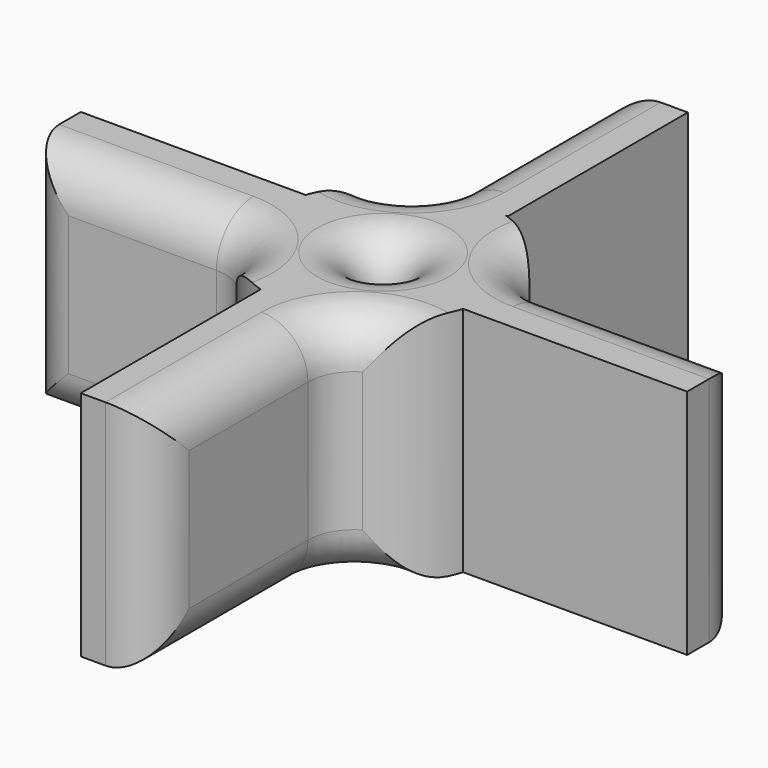
from build123d import *

# Parameters (mm, degrees)
F0_R         = 4.211
F0_W         = 0.5461883944
F0_H         = 48.4801451702
F1_DEPTH     = 25
F2_T1_DEPTH  = 50
F2_T3_DEPTH  = 100
F2_T5_DEPTH  = 67.0975783302
F2_T7_DEPTH  = 67.2386600166
F2_T9_DEPTH  = 67.0975783302
F2_T11_DEPTH = 66.9249549756
F2_T18_ANGLE = 202.5983722588
F2_T20_ANGLE = 202.5983722588
F2_T22_ANGLE = 202.6248548609
F2_T24_ANGLE = 202.6248548609
F2_T26_ANGLE = 201.5951809175
F2_T28_ANGLE = 201.5951809175
F2_T30_ANGLE = 202.6248548609
F2_T32_ANGLE = 202.6248548609


# Not quite as in the source:
# - a fillet or chamfer that OpenCascade refuses, or shapes differently, is made with other operations: its cross-section is extruded or revolved along the edge and cut away or added


with BuildPart() as f1:
    # F0 (on Top) → F1 (new body, symmetric)
    with BuildSketch(Plane.XY):
        with BuildLine():
            Line((7.6582201656, -71.9089287116), (7.6582201656, -23.4287835415))
            ThreePointArc((7.6582201656, -23.4287835415), (17.4241101733, -17.4343516945), (23.4242794808, -7.6719857367))
            Line((23.4242794808, -7.6719857367), (71.7281472729, -7.6719857367))
            Line((71.7281472729, -7.6719857367), (71.7281472729, 8.1906429889))
            Line((71.7281472729, 8.1906429889), (23.2480021027, 8.1906429889))
            ThreePointArc((23.2480021027, 8.1906429889), (17.2293028181, 17.6268930541), (7.6582201656, 23.4287835415))
            Line((7.6582201656, 23.4287835415), (7.6582201656, 71.9089287116))
            Line((7.6582201656, 71.9089287116), (-7.6582201656, 71.9089287116))
            Line((-7.6582201656, 71.9089287116), (-7.6582201656, 23.4287835415))
            ThreePointArc((-7.6582201656, 23.4287835415), (-17.2293028181, 17.6268930541), (-23.2480021027, 8.1906429889))
            Line((-23.2480021027, 8.1906429889), (-71.7281472729, 8.1906429889))
            Line((-71.7281472729, 8.1906429889), (-71.7281472729, -7.6719857367))
            Line((-71.7281472729, -7.6719857367), (-23.4242794808, -7.6719857367))
            ThreePointArc((-23.4242794808, -7.6719857367), (-17.4241101733, -17.4343516945), (-7.6582201656, -23.4287835415))
            Line((-7.6582201656, -23.4287835415), (-7.6582201656, -71.9089287116))
            Line((-7.6582201656, -71.9089287116), (7.6582201656, -71.9089287116))
        make_face()
        Circle(F0_R, mode=Mode.SUBTRACT)
        with Locations((7.9313143628, 47.6688561266)):
            Rectangle(F0_W, F0_H)
    extrude(amount=F1_DEPTH, both=True)

    # F2: fillet of radius 10 on 18 edges, made by hand

    # F2_s2 → F2_t1 (join)
    with BuildSketch(Plane.XY.offset(-25)):
        with BuildLine():
            ThreePointArc((-12.5618550278, 21.2074522892), (-8.9701924441, 24.8597673709), (-7.6582201656, 29.8113503815))
            Line((-7.6582201656, 29.8113503815), (-7.6582201656, 23.4287835415))
            ThreePointArc((-7.6582201656, 23.4287835415), (-10.170862222, 22.4523895387), (-12.5618550278, 21.2074522892))
        make_face()
        with BuildLine():
            ThreePointArc((20.9784825584, 12.9406145096), (24.6161046934, 9.458510237), (29.4894872562, 8.1906429889))
            Line((29.4894872562, 8.1906429889), (23.2480021027, 8.1906429889))
            ThreePointArc((23.2480021027, 8.1906429889), (22.2404146484, 10.6263912316), (20.9784825584, 12.9406145096))
        make_face()
        with BuildLine():
            ThreePointArc((12.5618550278, -21.2074522892), (8.9701924441, -24.8597673709), (7.6582201656, -29.8113503815))
            Line((7.6582201656, -29.8113503815), (7.6582201656, -23.4287835415))
            ThreePointArc((7.6582201656, -23.4287835415), (10.170862222, -22.4523895387), (12.5618550278, -21.2074522892))
        make_face()
        with BuildLine():
            ThreePointArc((-21.2016487218, -12.5716476969), (-24.8536155677, -8.9828148787), (-29.8031922973, -7.6719857367))
            Line((-29.8031922973, -7.6719857367), (-23.4242794808, -7.6719857367))
            ThreePointArc((-23.4242794808, -7.6719857367), (-22.4470496684, -10.1826418734), (-21.2016487218, -12.5716476969))
        make_face()
    extrude(amount=F2_T1_DEPTH)

    # F2_s4 → F2_t3 (cut)
    with BuildSketch(Plane.XY.offset(-50)):
        with BuildLine():
            ThreePointArc((2.3417798344, 71.9089287116), (-4.7292879775, 68.9799965235), (-7.6582201656, 61.9089287116))
            Line((-7.6582201656, 61.9089287116), (-7.6582201656, 71.9089287116))
            Line((-7.6582201656, 71.9089287116), (2.3417798344, 71.9089287116))
        make_face()
        with BuildLine():
            ThreePointArc((71.7281472729, -1.8093570111), (68.7992150847, 5.2617108008), (61.7281472729, 8.1906429889))
            Line((61.7281472729, 8.1906429889), (71.7281472729, 8.1906429889))
            Line((71.7281472729, 8.1906429889), (71.7281472729, -1.8093570111))
        make_face()
        with BuildLine():
            ThreePointArc((-2.3417798344, -71.9089287116), (4.7292879775, -68.9799965235), (7.6582201656, -61.9089287116))
            Line((7.6582201656, -61.9089287116), (7.6582201656, -71.9089287116))
            Line((7.6582201656, -71.9089287116), (-2.3417798344, -71.9089287116))
        make_face()
        with BuildLine():
            ThreePointArc((-71.7281472729, 2.3280142633), (-68.7992150847, -4.7430535485), (-61.7281472729, -7.6719857367))
            Line((-61.7281472729, -7.6719857367), (-71.7281472729, -7.6719857367))
            Line((-71.7281472729, -7.6719857367), (-71.7281472729, 2.3280142633))
        make_face()
    extrude(amount=F2_T3_DEPTH, mode=Mode.SUBTRACT)

    # F2_s6 → F2_t5 (cut)
    with BuildSketch(Plane.XZ.offset(-96.9089287116)):
        with BuildLine():
            ThreePointArc((2.3417798344, -25), (-4.7292879775, -22.0710678119), (-7.6582201656, -15))
            Line((-7.6582201656, -15), (-7.6582201656, -25))
            Line((-7.6582201656, -25), (2.3417798344, -25))
        make_face()
        with BuildLine():
            ThreePointArc((2.3417798344, 25), (-4.7292879775, 22.0710678119), (-7.6582201656, 15))
            Line((-7.6582201656, 15), (-7.6582201656, 25))
            Line((-7.6582201656, 25), (2.3417798344, 25))
        make_face()
    extrude(amount=F2_T5_DEPTH, mode=Mode.SUBTRACT)

    # F2_s8 → F2_t7 (cut)
    with BuildSketch(Plane.YZ.offset(29.4894872562)):
        with BuildLine():
            ThreePointArc((-1.8093570111, -25), (5.2617108008, -22.0710678119), (8.1906429889, -15))
            Line((8.1906429889, -15), (8.1906429889, -25))
            Line((8.1906429889, -25), (-1.8093570111, -25))
        make_face()
        with BuildLine():
            ThreePointArc((-1.8093570111, 25), (5.2617108008, 22.0710678119), (8.1906429889, 15))
            Line((8.1906429889, 15), (8.1906429889, 25))
            Line((8.1906429889, 25), (-1.8093570111, 25))
        make_face()
    extrude(amount=F2_T7_DEPTH, mode=Mode.SUBTRACT)

    # F2_s10 → F2_t9 (cut)
    with BuildSketch(Plane.XZ.offset(29.8113503815)):
        with BuildLine():
            ThreePointArc((-2.3417798344, -25), (4.7292879775, -22.0710678119), (7.6582201656, -15))
            Line((7.6582201656, -15), (7.6582201656, -25))
            Line((7.6582201656, -25), (-2.3417798344, -25))
        make_face()
        with BuildLine():
            ThreePointArc((-2.3417798344, 25), (4.7292879775, 22.0710678119), (7.6582201656, 15))
            Line((7.6582201656, 15), (7.6582201656, 25))
            Line((7.6582201656, 25), (-2.3417798344, 25))
        make_face()
    extrude(amount=F2_T9_DEPTH, mode=Mode.SUBTRACT)

    # F2_s12 → F2_t11 (cut)
    with BuildSketch(Plane.YZ.offset(-96.7281472729)):
        with BuildLine():
            ThreePointArc((2.3280142633, -25), (-4.7430535485, -22.0710678119), (-7.6719857367, -15))
            Line((-7.6719857367, -15), (-7.6719857367, -25))
            Line((-7.6719857367, -25), (2.3280142633, -25))
        make_face()
        with BuildLine():
            ThreePointArc((2.3280142633, 25), (-4.7430535485, 22.0710678119), (-7.6719857367, 15))
            Line((-7.6719857367, 15), (-7.6719857367, 25))
            Line((-7.6719857367, 25), (2.3280142633, 25))
        make_face()
    extrude(amount=F2_T11_DEPTH, mode=Mode.SUBTRACT)

    # F2_s13 → F2_t14 (revolve, cut)
    with BuildSketch(Plane.XZ):
        with BuildLine():
            ThreePointArc((14.211, -25), (7.1399321881, -22.0710678119), (4.211, -15))
            Line((4.211, -15), (4.211, -25))
            Line((4.211, -25), (14.211, -25))
        make_face()
    revolve(axis=Axis((0, 0, -25), (0, 0, 1)), mode=Mode.SUBTRACT)

    # F2_s15 → F2_t16 (revolve, cut)
    with BuildSketch(Plane.XZ):
        with BuildLine():
            ThreePointArc((14.211, 25), (7.1399321881, 22.0710678119), (4.211, 15))
            Line((4.211, 15), (4.211, 25))
            Line((4.211, 25), (14.211, 25))
        make_face()
    revolve(axis=Axis((0, 0, 25), (0, 0, 1)), mode=Mode.SUBTRACT)

    # F2_s17 → F2_t18 (revolve, cut)
    with BuildSketch(Plane(origin=(-19.132963154, 7.963646146, 0), x_dir=(0, 0, 1), z_dir=(-0.9232211344, 0.3842690946, 0))):
        with BuildLine():
            ThreePointArc((25, -47.7675964389), (22.0710678119, -40.696528627), (15, -37.7675964389))
            Line((15, -37.7675964389), (25, -37.7675964389))
            Line((25, -37.7675964389), (25, -47.7675964389))
        make_face()
    revolve(axis=Axis((-29.8031922972, -17.6719857367, 25), (0, 0, 1)), revolution_arc=F2_T18_ANGLE, mode=Mode.SUBTRACT)

    # F2_s19 → F2_t20 (revolve, cut)
    with BuildSketch(Plane(origin=(-19.132963154, 7.963646146, 0), x_dir=(0, 0, 1), z_dir=(-0.9232211344, 0.3842690946, 0))):
        with BuildLine():
            ThreePointArc((-25, -47.7675964389), (-22.0710678119, -40.696528627), (-15, -37.7675964389))
            Line((-15, -37.7675964389), (-25, -37.7675964389))
            Line((-25, -37.7675964389), (-25, -47.7675964389))
        make_face()
    revolve(axis=Axis((-29.8031922972, -17.6719857367, -25), (0, 0, 1)), revolution_arc=F2_T20_ANGLE, mode=Mode.SUBTRACT)

    # F2_s21 → F2_t22 (revolve, cut)
    with BuildSketch(Plane(origin=(-7.9724845558, -19.1292702646, 0), x_dir=(0, 0, 1), z_dir=(-0.3846957743, -0.9230434233, 0))):
        with BuildLine():
            ThreePointArc((25, -47.7676045084), (22.0710678119, -40.6965366966), (15, -37.7676045084))
            Line((15, -37.7676045084), (25, -37.7676045084))
            Line((25, -37.7676045084), (25, -47.7676045084))
        make_face()
    revolve(axis=Axis((17.6582201656, -29.8113503815, 25), (0, 0, 1)), revolution_arc=F2_T22_ANGLE, mode=Mode.SUBTRACT)

    # F2_s23 → F2_t24 (revolve, cut)
    with BuildSketch(Plane(origin=(-7.9724845558, -19.1292702646, 0), x_dir=(0, 0, 1), z_dir=(-0.3846957743, -0.9230434233, 0))):
        with BuildLine():
            ThreePointArc((-25, -47.7676045084), (-22.0710678119, -40.6965366966), (-15, -37.7676045084))
            Line((-15, -37.7676045084), (-25, -37.7676045084))
            Line((-25, -37.7676045084), (-25, -47.7676045084))
        make_face()
    revolve(axis=Axis((17.6582201656, -29.8113503815, -25), (0, 0, 1)), revolution_arc=F2_T24_ANGLE, mode=Mode.SUBTRACT)

    # F2_s25 → F2_t26 (revolve, cut)
    with BuildSketch(Plane(origin=(19.2698363003, -7.6275931455, 0), x_dir=(0, 0, 1), z_dir=(0.9298074451, -0.3680463489, 0))):
        with BuildLine():
            ThreePointArc((25, -47.7672933998), (22.0710678119, -40.6962255879), (15, -37.7672933998))
            Line((15, -37.7672933998), (25, -37.7672933998))
            Line((25, -37.7672933998), (25, -47.7672933998))
        make_face()
    revolve(axis=Axis((29.4894872562, 18.1906429889, 25), (0, 0, 1)), revolution_arc=F2_T26_ANGLE, mode=Mode.SUBTRACT)

    # F2_s27 → F2_t28 (revolve, cut)
    with BuildSketch(Plane(origin=(19.2698363003, -7.6275931455, 0), x_dir=(0, 0, 1), z_dir=(0.9298074451, -0.3680463489, 0))):
        with BuildLine():
            ThreePointArc((-25, -47.7672933998), (-22.0710678119, -40.6962255879), (-15, -37.7672933998))
            Line((-15, -37.7672933998), (-25, -37.7672933998))
            Line((-25, -37.7672933998), (-25, -47.7672933998))
        make_face()
    revolve(axis=Axis((29.4894872562, 18.1906429889, -25), (0, 0, 1)), revolution_arc=F2_T28_ANGLE, mode=Mode.SUBTRACT)

    # F2_s29 → F2_t30 (revolve, cut)
    with BuildSketch(Plane(origin=(7.9724845558, 19.1292702646, 0), x_dir=(0, 0, 1), z_dir=(0.3846957743, 0.9230434233, 0))):
        with BuildLine():
            ThreePointArc((25, -47.7676045084), (22.0710678119, -40.6965366966), (15, -37.7676045084))
            Line((15, -37.7676045084), (25, -37.7676045084))
            Line((25, -37.7676045084), (25, -47.7676045084))
        make_face()
    revolve(axis=Axis((-17.6582201656, 29.8113503815, 25), (0, 0, 1)), revolution_arc=F2_T30_ANGLE, mode=Mode.SUBTRACT)

    # F2_s31 → F2_t32 (revolve, cut)
    with BuildSketch(Plane(origin=(7.9724845558, 19.1292702646, 0), x_dir=(0, 0, 1), z_dir=(0.3846957743, 0.9230434233, 0))):
        with BuildLine():
            ThreePointArc((-25, -47.7676045084), (-22.0710678119, -40.6965366966), (-15, -37.7676045084))
            Line((-15, -37.7676045084), (-25, -37.7676045084))
            Line((-25, -37.7676045084), (-25, -47.7676045084))
        make_face()
    revolve(axis=Axis((-17.6582201656, 29.8113503815, -25), (0, 0, 1)), revolution_arc=F2_T32_ANGLE, mode=Mode.SUBTRACT)


solid = f1.part
